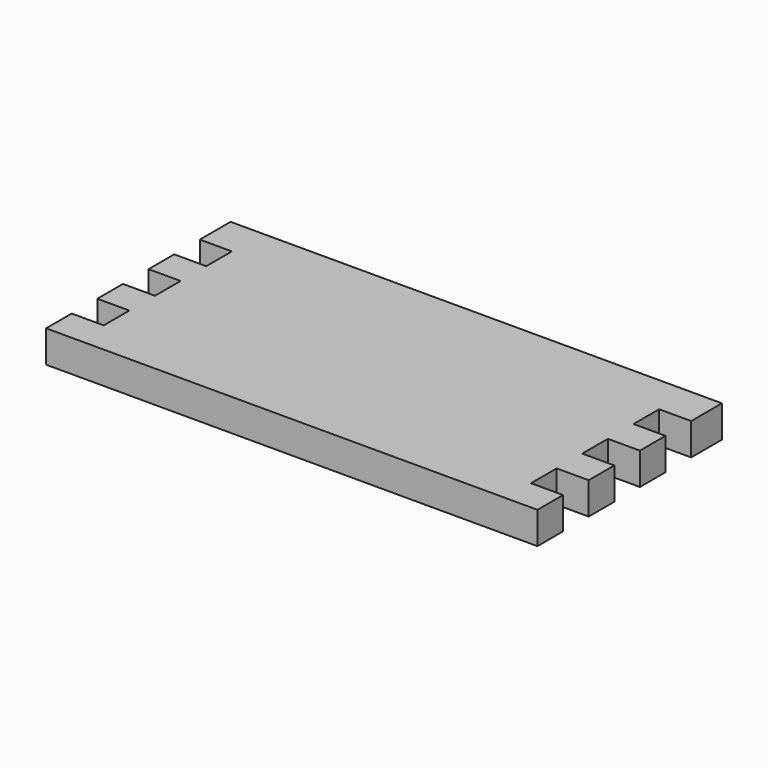
from build123d import *

# Parameters (mm, degrees)
F0_W     = 10
F0_H     = 10
F1_DEPTH = 10


# Not quite as in the source:
# - a feature names something its author has since deleted; it is built from what else it names


with BuildPart() as f1:
    # F0 (on Top) → F1 (new body)
    with BuildSketch(Plane.XY):
        Polygon((-2.2346749902, 36.9413525529), (-135.6346749902, 36.9413525529), (-135.6346749902, 26.9413525529), (-135.6346749902, 16.9413525529), (-135.6346749902, 6.9413525529), (-135.6346749902, -3.0586474471), (-135.6346749902, -13.0586474471), (-135.6346749902, -23.0586474471), (-135.6346749902, -33.0586474471), (-2.2346749902, -33.0586474471), (-2.2346749902, -23.0586474471), (-2.2346749902, -13.0586474471), (-2.2346749902, -3.0586474471), (-2.2346749902, 6.9413525529), (-2.2346749902, 16.9413525529), (-2.2346749902, 26.9413525529), align=None)
        with Locations((-140.6346749902, 31.9413525529)):
            Rectangle(F0_W, F0_H)
        with Locations((-140.6346749902, 11.9413525529)):
            Rectangle(F0_W, F0_H)
        with Locations((-140.6346749902, -8.0586474471)):
            Rectangle(F0_W, F0_H)
        with Locations((-140.6346749902, -28.0586474471)):
            Rectangle(F0_W, F0_H)
        with Locations((2.7653250098, 31.9413525529)):
            Rectangle(F0_W, F0_H)
        with Locations((2.7653250098, 11.9413525529)):
            Rectangle(F0_W, F0_H)
        with Locations((2.7653250098, -8.0586474471)):
            Rectangle(F0_W, F0_H)
        with Locations((2.7653250098, -28.0586474471)):
            Rectangle(F0_W, F0_H)
        Polygon((-145.6346749902, 38.9413525529), (-145.6346749902, 36.9413525529), (-135.6346749902, 36.9413525529), (-2.2346749902, 36.9413525529), (7.7653250098, 36.9413525529), (7.7653250098, 38.9413525529), align=None)
    extrude(amount=F1_DEPTH)


solid = f1.part
